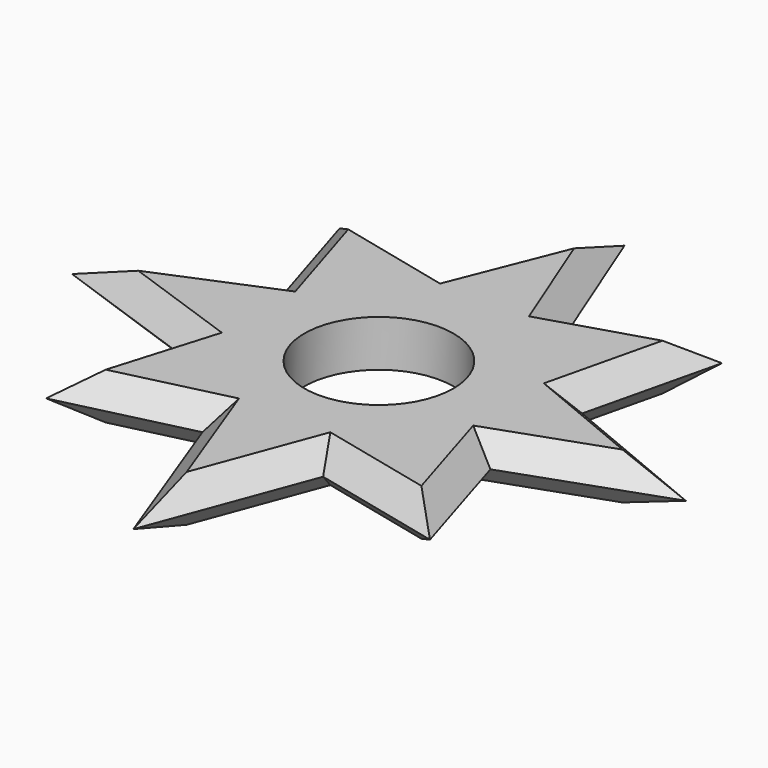
from build123d import *

# Parameters (mm, degrees)
F0_R     = 11.0998
F1_DEPTH = 6.9342
F2_SIZE  = 3.4671
F3_SIZE  = 3.46709
F5_DEPTH = 6.9342
F6_SIZE  = 3.46709


# Not quite as in the source:
# - a fillet or chamfer is up to 0.001 mm smaller than in the source, because OpenCascade refuses the exact size


with BuildPart() as f1:
    # F0 (on Top) → F1 (new body)
    with BuildSketch(Plane.XY):
        Polygon((12.7, 13.7528510513), (0, 45.72), (-12.7, 13.7528510513), (-45.72, 0), (-12.7, -11.6471489487), (0, -45.72), (12.7, -11.6471489487), (45.72, 0), align=None)
        Circle(F0_R, mode=Mode.SUBTRACT)
    extrude(amount=F1_DEPTH)

    # F2
    f2_edges = [f1.edges().sort_by_distance(p)[0] for p in [
        (6.35, -28.683574, 6.9342),
        (29.21, -5.823574, 6.9342),
        (-29.21, -5.823574, 6.9342),
        (-6.35, 29.736426, 6.9342),
        (-29.21, 6.876426, 6.9342),
        (6.35, 29.736426, 6.9342),
        (29.21, 6.876426, 6.9342),
        (-6.35, -28.683574, 6.9342),
    ]]
    chamfer(f2_edges, length=F2_SIZE)

    # F3 (size 3.4671 in the source; OpenCascade refuses exactly that, so slightly less here)
    f3_edges = [f1.edges().sort_by_distance(p)[0] for p in [
        (6.35, -28.683574, 0),
        (29.21, -5.823574, 0),
        (-29.21, -5.823574, 0),
        (-6.35, -28.683574, 0),
        (6.35, 29.736426, 0),
        (29.21, 6.876426, 0),
        (-29.21, 6.876426, 0),
        (-6.35, 29.736426, 0),
    ]]
    chamfer(f3_edges, length=F3_SIZE)

    # F4 (on face) → F5 (join)
    with BuildSketch(Plane.XY.offset(6.9342)):
        Polygon((-5.3285628953, 22.9169632653), (-28.5960960526, 28.4347391196), (-10.0175652565, 11.1142831944), align=None)
        Polygon((-28.5960960526, 28.4347391196), (-21.7413331227, 6.2313264038), (-10.0175652565, 11.1142831944), align=None)
        Polygon((27.3380211817, 29.6928139905), (5.3285628953, 22.9169632653), (10.0175652565, 11.1142831944), align=None)
        Polygon((27.3380211817, 29.6928139905), (10.0175652565, 11.1142831944), (21.7413331227, 6.2313264038), align=None)
        Polygon((10.0175516395, -8.916864886), (5.5819678365, -20.8171000234), (28.5960824356, -26.2373208112), align=None)
        Polygon((-5.5819678365, -20.8171000234), (-10.0175516395, -8.916864886), (-28.504862756, -26.3346525665), align=None)
        Polygon((-10.0175516395, -8.916864886), (-21.9943219535, -4.6922971158), (-28.504862756, -26.3346525665), align=None)
        Polygon((21.9943219535, -4.6922971158), (10.0175516395, -8.916864886), (28.5960824356, -26.2373208112), align=None)
    extrude(amount=-F5_DEPTH)

    # F6 (size 3.4671 in the source; OpenCascade refuses exactly that, so slightly less here)
    f6_edges = [f1.edges().sort_by_distance(p)[0] for p in [
        (17.089025, -23.52721, 6.9342),
        (25.295202, -15.464809, 6.9342),
        (24.539677, 17.96207, 6.9342),
        (-17.043415, -23.575876, 6.9342),
        (-25.249592, -15.513475, 6.9342),
        (-25.168715, 17.333033, 6.9342),
        (-16.962329, 25.675851, 6.9342),
        (16.333292, 26.304889, 6.9342),
        (24.539678, 17.962075, 0),
        (25.295204, -15.464814, 0),
        (17.08903, -23.527212, 0),
        (-17.04342, -23.575877, 0),
        (16.333297, 26.30489, 0),
        (-16.962334, 25.675852, 0),
        (-25.168716, 17.333038, 0),
        (-25.249594, -15.51348, 0),
    ]]
    chamfer(f6_edges, length=F6_SIZE)


solid = f1.part
